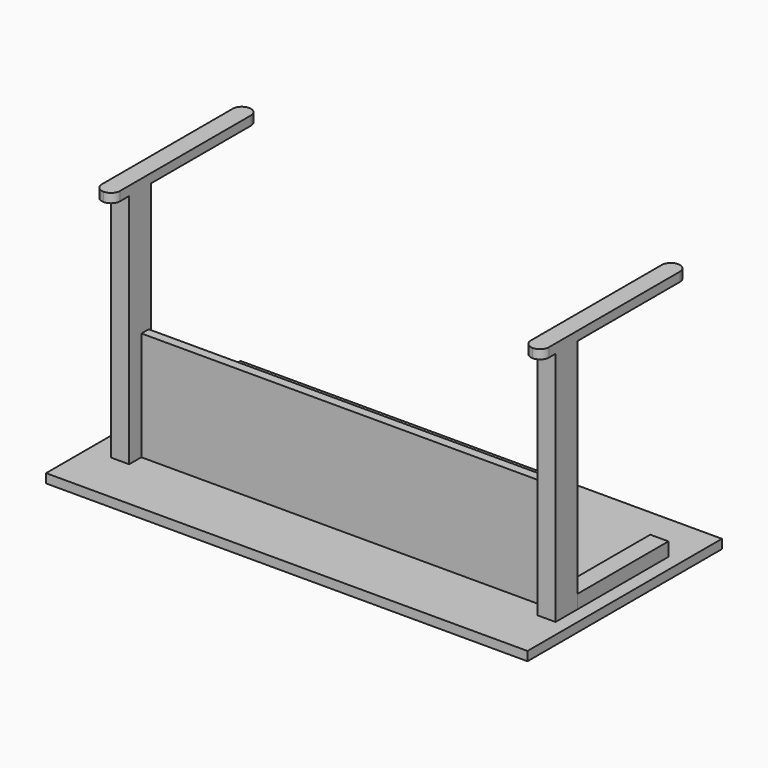
from build123d import *

# Parameters (mm, degrees)
F0_W      = 1346.2
F0_H      = 679.45
F1_DEPTH  = 25.4
F3_W      = 50.8
F3_H      = 317.5
F4_W      = 50.8
F4_H      = 317.5
F5_DEPTH  = 38.1
F7_W      = 50.8
F7_H      = 76.2
F6_W      = 50.8
F6_H      = 76.2
F8_DEPTH  = 660.4
F10_W     = 50.8
F10_H     = 508
F9_W      = 50.8
F9_H      = 508
F11_DEPTH = 25.4
F12_R     = 25.39999
F13_R     = 25.4
F14_W     = 1143.3658423165
F14_H     = 25.4
F15_DEPTH = 304.8


# Not quite as in the source:
# - a fillet or chamfer is up to 0.001 mm smaller than in the source, because OpenCascade refuses the exact size


with BuildPart() as f1:
    # F0 (on Top) → F1 (new body)
    with BuildSketch(Plane.XY):
        with Locations((149.0168645364, 3.430750221)):
            Rectangle(F0_W, F0_H)
    extrude(amount=F1_DEPTH)

    # F3 (on face) + F4 (on face) → F5 (join)
    with BuildSketch(Plane.XY.offset(25.4)):
        with Locations((-433.5340384189, 44.705750221)):
            Rectangle(F3_W, F3_H)
    with BuildSketch(Plane.XY.offset(25.4)):
        with Locations((758.8858046625, 44.705750221)):
            Rectangle(F4_W, F4_H)
    extrude(amount=F5_DEPTH)

    # F7 (on face) + F6 (on face) → F8 (join)
    with BuildSketch(Plane.XY.offset(25.4)):
        with Locations((-433.9627325535, -152.2812862285)):
            Rectangle(F7_W, F7_H)
    with BuildSketch(Plane.XY.offset(25.4)):
        with Locations((758.9168250561, -152.9612190686)):
            Rectangle(F6_W, F6_H)
    extrude(amount=F8_DEPTH)

    # F10 (on face) + F9 (on face) → F11 (join)
    with BuildSketch(Plane.XY.offset(685.8)):
        with Locations((758.9168250561, 14.9119266272)):
            Rectangle(F10_W, F10_H)
    with BuildSketch(Plane.XY.offset(685.8)):
        with Locations((-433.9627325535, 6.5043487549)):
            Rectangle(F9_W, F9_H)
    extrude(amount=F11_DEPTH)

    # F12 (radius 25.4 in the source; OpenCascade refuses exactly that, so slightly less here)
    f12_edges = [f1.edges().sort_by_distance(p)[0] for p in [
        (-459.362733, 260.504349, 698.5),
        (-408.562733, 260.504349, 698.5),
        (733.516825, 268.911927, 698.5),
        (784.316825, 268.911927, 698.5),
        (-459.362733, -247.495651, 698.5),
        (-408.562733, -247.495651, 698.5),
        (733.516825, -239.088073, 698.5),
    ]]
    fillet(f12_edges, radius=F12_R)

    # F13
    f13_edges = [f1.edges().sort_by_distance(p)[0] for p in [
        (784.316825, -239.088073, 698.5),
    ]]
    fillet(f13_edges, radius=F13_R)

    # F14 (on face) → F15 (join)
    with BuildSketch(Plane.XY.offset(25.4)):
        with Locations((163.3197753559, -135.036409986)):
            Rectangle(F14_W, F14_H)
    extrude(amount=F15_DEPTH)


solid = f1.part
